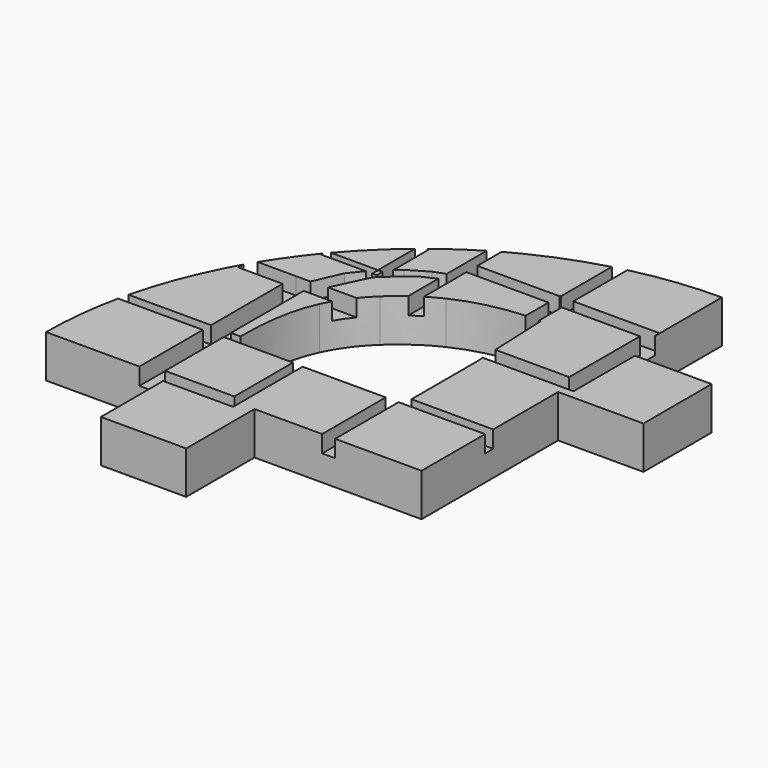
from build123d import *

# Parameters (mm, degrees)
F1_W     = 9.5782261753
F1_H     = 9.891791337
F1_H_2   = 10.108208663
F1_W_2   = 10
F1_H_3   = 10
F2_DEPTH = 5
F3_W     = 10.1701691747
F3_H     = 1.1901259422
F3_W_2   = 2.3802500218
F3_W_3   = 1.1901250109
F3_H_2   = 0.8006438729
F3_H_3   = 10.4947462678
F3_W_4   = 5.1932781935
F3_H_4   = 1.9474774599
F3_W_5   = 1.1901259422
F3_H_5   = 8.5062488797
F3_W_6   = 9.7373928875
F3_W_7   = 1.514704898
F3_H_6   = 9.3068927526
F3_W_8   = 10.1330708712
F3_H_7   = 1.6025230289
F3_W_9   = 9.0882331133
F3_H_8   = 3.835350275
F3_W_10  = 1.0448377579
F3_H_9   = 8.595854044
F3_W_11  = 1.0108357528
F3_W_12  = 1.0278367554
F3_H_10  = 0.8937604725
F4_DEPTH = 25
F5_W     = 8.1058442593
F5_H     = 1.9299630076
F5_W_2   = 1.5439689159
F5_W_3   = 1.5439717099
F5_H_2   = 11.9657684118
F5_W_4   = 10.3005599231
F5_H_3   = 1.0513318703
F6_DEPTH = 25


# Not quite as in the source:
# - a feature names something its author has since deleted; it is built from what else it names


with BuildPart() as f2:
    # F1 (on Top) → F2 (new body)
    with BuildSketch(Plane.XY):
        with Locations((-4.7891130877, 4.9458956685)):
            Rectangle(F1_W, F1_H)
        Polygon((-10, 0), (-9.5782261753, 0), (-9.5782261753, 9.891791337), (-19.5782261753, 9.891791337), (-19.5782261753, 0), align=None)
        with Locations((-4.7891130877, 14.9458956685)):
            Rectangle(F1_W, F1_H_2)
        Polygon((0, 30), (0, 20), (0.4217738247, 20), (10, 20), (10, 30), align=None)
        Polygon((-9.5782261753, 20), (0, 20), (0, 30), (-10.0065707871, 30), align=None)
        with Locations((-24.5782261753, 4.9458956685)):
            Rectangle(F1_W_2, F1_H)
        with Locations((-24.5782261753, -5)):
            Rectangle(F1_W_2, F1_H_3)
        with BuildLine():
            Line((-10.0065707871, 30), (0, 30))
            Line((0, 30), (0, 44))
            ThreePointArc((0, 44), (-5.0363871882, 43.7108087787), (-10.0065707871, 42.8470365496))
            Line((-10.0065707871, 42.8470365496), (-10.0065707871, 30))
        make_face()
        with BuildLine():
            Line((-44, 0), (-29.5782261753, 0))
            Line((-29.5782261753, 0), (-29.5782261753, 9.891791337))
            add(Edge.make_bspline(
                [(-29.5782261753, 9.891791337), (-29.5956822452, 12.6865898133), (-29.4779762378, 16.6539770733), (-27.9306023487, 20)],
                knots=[0, 0, 0, 0, 0.3288616787, 0.3288616787, 0.3288616787, 0.3288616787], degree=3))
            Line((-27.9306023487, 20), (-39.1918358845, 20))
            ThreePointArc((-39.1918358845, 20), (-42.7810751321, 10.2849215136), (-44, 0))
        make_face()
        with BuildLine():
            add(Edge.make_bspline(
                [(-19.5782261753, 28.0459611928), (-16.4208018887, 29.540455447), (-13.1162348053, 30), (-10.0065707871, 30)],
                knots=[0.678814496, 0.678814496, 0.678814496, 0.678814496, 1, 1, 1, 1], degree=3))
            Line((-10.0065707871, 30), (-10.0065707871, 42.8470365496))
            ThreePointArc((-10.0065707871, 42.8470365496), (-14.8922224071, 41.4031606496), (-19.5782261753, 39.4042264209))
            Line((-19.5782261753, 39.4042264209), (-19.5782261753, 28.0459611928))
        make_face()
        with BuildLine():
            add(Edge.make_bspline(
                [(-24.5782261753, 24.6040217078), (-23.0917294817, 26.0318138691), (-21.358363516, 27.2033740757), (-19.5782261753, 28.0459611928)],
                knots=[0.497731988, 0.497731988, 0.497731988, 0.497731988, 0.678814496, 0.678814496, 0.678814496, 0.678814496], degree=3))
            Line((-19.5782261753, 28.0459611928), (-19.5782261753, 39.4042264209))
            ThreePointArc((-19.5782261753, 39.4042264209), (-23.9356591488, 36.9199704918), (-27.9820429197, 33.9559313529))
            Line((-27.9820429197, 33.9559313529), (-24.5782261753, 24.6040217078))
        make_face()
        with BuildLine():
            Line((-39.1918358845, 20), (-27.9306023487, 20))
            add(Edge.make_bspline(
                [(-27.9306023487, 20), (-27.136026622, 21.7181811177), (-25.9644735778, 23.2725198056), (-24.5782261753, 24.6040217078)],
                knots=[0.3288616787, 0.3288616787, 0.3288616787, 0.3288616787, 0.497731988, 0.497731988, 0.497731988, 0.497731988], degree=3))
            Line((-24.5782261753, 24.6040217078), (-33.9336129947, 28.00910404))
            ThreePointArc((-33.9336129947, 28.00910404), (-36.7813710365, 24.148100229), (-39.1918358845, 20))
        make_face()
        with BuildLine():
            Line((-33.9336129947, 28.00910404), (-24.5782261753, 24.6040217078))
            Line((-24.5782261753, 24.6040217078), (-27.9820429197, 33.9559313529))
            ThreePointArc((-27.9820429197, 33.9559313529), (-31.1002942205, 31.1250975806), (-33.9336129947, 28.00910404))
        make_face()
    extrude(amount=F2_DEPTH)

    # F3 (on offset) → F4 (cut)
    with BuildSketch(Plane.XY.offset(3)):
        Polygon((-33.0700390041, 9.3068927526), (-33.0700390041, 0), (-31.8799139932, 0), (-31.8799139932, 0.8006438729), (-30.6897889823, 0.8006438729), (-30.6897889823, 9.3068927526), align=None)
        with Locations((-38.1551235914, 9.9019557238)):
            Rectangle(F3_W, F3_H)
        with Locations((-31.8799139932, 9.9019557238)):
            Rectangle(F3_W_2, F3_H)
        with Locations((-31.2848514877, 0.4003219365)):
            Rectangle(F3_W_3, F3_H_2)
        Polygon((-30.6897889823, 0), (-31.8799139932, 0), (-31.8799139932, -0.8824482211), (-21.3851686567, -0.8824482211), (-21.3851686567, 0), (-22.5752945989, 0), (-22.5752945989, 0.8006438729), (-30.6897889823, 0.8006438729), align=None)
        with Locations((-31.8799139932, 15.7443918288)):
            Rectangle(F3_W_2, F3_H_3)
        with Locations((-35.6666781008, 21.9655036926)):
            Rectangle(F3_W_4, F3_H_4)
        Polygon((-33.0700390041, 22.9392424226), (-33.0700390041, 20.9917649627), (-30.6897889823, 20.9917649627), (-30.6897889823, 22.9392424226), (-31.3607603312, 22.9392424226), align=None)
        with Locations((-21.9802316278, 5.0537683128)):
            Rectangle(F3_W_5, F3_H_5)
        with Locations((-21.9802316278, 9.9019557238)):
            Rectangle(F3_W_5, F3_H)
        with Locations((-21.9802316278, 0.4003219365)):
            Rectangle(F3_W_5, F3_H_2)
        with Locations((-16.516472213, 9.9019557238)):
            Rectangle(F3_W_6, F3_H)
        Polygon((-29.9641676247, 26.1324569583), (-31.3607603312, 22.9392424226), (-30.6897889823, 22.9392424226), (-29.4176749885, 22.9392424226), (-28.3854100853, 25.160914287), (-27.413867414, 27.1647218615), (-25.7743895054, 28.682757169), (-24.2563541979, 29.8971850425), (-22.5752945989, 30.6865628809), (-22.5752945989, 31.9009907544), (-23.8920263946, 31.41522035), (-26.1387173086, 30.0793480128), (-26.8673747778, 29.40273819), (-26.8673747778, 27.7112144977), (-27.413867414, 27.7112144977), (-27.9603600502, 27.7112144977), (-28.6890175194, 27.7112144977), align=None)
        with Locations((-10.8904233202, 4.6534463763)):
            Rectangle(F3_W_7, F3_H_6)
        with Locations((-10.8904233202, 9.9019557238)):
            Rectangle(F3_W_7, F3_H)
        Polygon((-22.5752945989, 30.6865628809), (-22.5752945989, 22.9392424226), (-21.3851686567, 22.9392424226), (-21.3851686567, 33.2975834608), (-22.5752945989, 33.2975834608), (-22.5752945989, 31.9009907544), align=None)
        with Locations((-10.8904233202, 15.7443918288)):
            Rectangle(F3_W_7, F3_H_3)
        with Locations((-5.0665354356, 9.9019557238)):
            Rectangle(F3_W_8, F3_H)
        Polygon((-27.9603600502, 28.3878243205), (-28.6890175194, 27.7112144977), (-27.9603600502, 27.7112144977), align=None)
        Polygon((-33.9717790484, 27.7112144977), (-28.6890175194, 27.7112144977), (-27.9603600502, 28.3878243205), (-27.9603600502, 28.5613127053), (-33.9717790484, 28.5613127053), align=None)
        with Locations((-10.8904233202, 21.9655036926)):
            Rectangle(F3_W_7, F3_H_4)
        Polygon((-27.9603600502, 28.5613127053), (-27.9603600502, 28.3878243205), (-27.7735262161, 28.5613127053), align=None)
        with Locations((-21.9802316278, 34.0988449752)):
            Rectangle(F3_W_5, F3_H_7)
        with Locations((-16.516472213, 34.0988449752)):
            Rectangle(F3_W_6, F3_H_7)
        with Locations((-5.5889543146, 21.9655036926)):
            Rectangle(F3_W_9, F3_H_4)
        Polygon((-27.413867414, 28.5613127053), (-27.413867414, 27.7112144977), (-26.8673747778, 27.7112144977), (-26.8673747778, 29.40273819), (-27.7735262161, 28.5613127053), align=None)
        Polygon((-27.9603600502, 34.6941761672), (-27.9603600502, 28.5613127053), (-27.7735262161, 28.5613127053), (-26.8673747778, 29.40273819), (-26.8673747778, 34.6941761672), align=None)
        with Locations((-21.9802316278, 36.8177816272)):
            Rectangle(F3_W_5, F3_H_8)
        with Locations((-10.8904233202, 34.0988449752)):
            Rectangle(F3_W_7, F3_H_7)
        with Locations((-0.522418879, 21.9655036926)):
            Rectangle(F3_W_10, F3_H_4)
        with Locations((-10.8904233202, 39.1980335116)):
            Rectangle(F3_W_7, F3_H_9)
        Polygon((-10.1330708712, 34.9001064897), (-10.1330708712, 33.2975834608), (-1.0448377579, 33.2975834608), (-1.0448377579, 34.1913439333), (-0.0170010026, 34.1913439333), (-0.0170010026, 34.9001064897), align=None)
        Polygon((-1.0448377579, 33.2975834608), (-1.0448377579, 22.9392424226), (0, 22.9392424226), (1.0108357528, 22.9392424226), (1.0108357528, 34.1913439333), (-0.0170010026, 34.1913439333), (-0.0170010026, 33.2975834608), align=None)
        with Locations((0.5054178764, 21.9655036926)):
            Rectangle(F3_W_11, F3_H_4)
        with Locations((-0.5309193803, 33.7444636971)):
            Rectangle(F3_W_12, F3_H_10)
    extrude(amount=F4_DEPTH, mode=Mode.SUBTRACT)

    # F5 (on offset) → F6 (cut)
    with BuildSketch(Plane.XY.offset(3)):
        with Locations((-26.8084984273, 22.0622615889)):
            Rectangle(F5_W, F5_H)
        with Locations((-21.9835918397, 22.0622615889)):
            Rectangle(F5_W_2, F5_H)
        Polygon((-11.7547893897, 23.0272430927), (-21.2116073817, 23.0272430927), (-21.2116073817, 21.0972800851), (-10.2108176798, 21.0972800851), (-10.2108176798, 23.0272430927), align=None)
        Polygon((-21.2116073817, 21.0972800851), (-22.7555762976, 21.0972800851), (-22.7555762976, 10.4401707649), (-22.7555762976, 9.3888388947), (-21.2116073817, 9.3888388947), align=None)
        with Locations((-10.9828035347, 29.0101272985)):
            Rectangle(F5_W_3, F5_H_2)
        with Locations((-27.9058562592, 9.9145048298)):
            Rectangle(F5_W_4, F5_H_3)
    extrude(amount=F6_DEPTH, mode=Mode.SUBTRACT)


solid = f2.part
